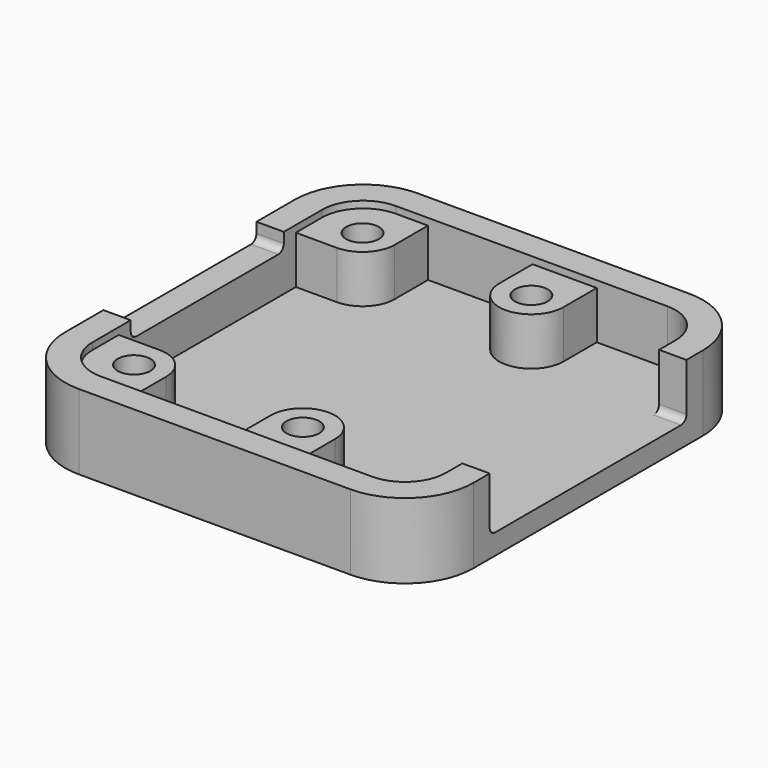
from build123d import *

# Parameters (mm, degrees)
F0_R      = 1.2
F1_DEPTH  = 1.5
F2_DEPTH  = 5
F3_DEPTH  = 5.5
F5_DEPTH  = 2
F7_DEPTH  = 2
F8_W      = 10
F8_H      = 5
F9_DEPTH  = 1
F10_R     = 1
F11_DEPTH = 5


# Not quite as in the source:
# - a feature names something its author has since deleted; it is built from what else it names


with BuildPart() as f1:
    # F0 (on Top) → F1 (new body)
    with BuildSketch(Plane.XY):
        with BuildLine():
            Line((14.9310000289, -10.5), (14.9310000289, 10.5))
            ThreePointArc((14.9310000289, 10.5), (13.4665339264, 14.0355339264), (9.931, 15.5000000289))
            Line((9.931, 15.5000000289), (-9.931, 15.5000000289))
            ThreePointArc((-9.931, 15.5000000289), (-13.4665339264, 14.0355339264), (-14.9310000289, 10.5))
            Line((-14.9310000289, 10.5), (-14.9310000289, -10.5))
            ThreePointArc((-14.9310000289, -10.5), (-13.4665339264, -14.0355339264), (-9.931, -15.5000000289))
            Line((-9.931, -15.5000000289), (9.931, -15.5000000289))
            ThreePointArc((9.931, -15.5000000289), (13.4665339264, -14.0355339264), (14.9310000289, -10.5))
        make_face()
        with BuildLine():
            Line((-9.931, 13.5000000289), (-7.581, 13.5000000289))
            Line((-7.581, 13.5000000289), (0.069, 13.5000000289))
            Line((0.069, 13.5000000289), (4.769, 13.5000000289))
            Line((4.769, 13.5000000289), (9.931, 13.5000000289))
            ThreePointArc((9.931, 13.5000000289), (12.052320364, 12.621320364), (12.9310000289, 10.5))
            Line((12.9310000289, 10.5), (12.9310000289, -10.5))
            ThreePointArc((12.9310000289, -10.5), (12.052320364, -12.621320364), (9.931, -13.5000000289))
            Line((9.931, -13.5000000289), (4.769, -13.5000000289))
            Line((4.769, -13.5000000289), (0.069, -13.5000000289))
            Line((0.069, -13.5000000289), (-7.581, -13.5000000289))
            Line((-7.581, -13.5000000289), (-9.931, -13.5000000289))
            ThreePointArc((-9.931, -13.5000000289), (-12.052320364, -12.621320364), (-12.9310000289, -10.5))
            Line((-12.9310000289, -10.5), (-12.9310000289, -8.1))
            Line((-12.9310000289, -8.1), (-12.9310000289, 8.1))
            Line((-12.9310000289, 8.1), (-12.9310000289, 10.5))
            ThreePointArc((-12.9310000289, 10.5), (-12.052320364, 12.621320364), (-9.931, 13.5000000289))
        make_face(mode=Mode.SUBTRACT)
        with BuildLine():
            ThreePointArc((4.769, -10.45), (2.419, -8.1), (0.069, -10.45))
            ThreePointArc((0.069, -10.45), (2.419, -12.8), (4.769, -10.45))
        make_face()
        with Locations((2.419, -10.45)):
            Circle(F0_R, mode=Mode.SUBTRACT)
        with BuildLine():
            ThreePointArc((4.769, 10.45), (2.419, 12.8), (0.069, 10.45))
            ThreePointArc((0.069, 10.45), (2.419, 8.1), (4.769, 10.45))
        make_face()
        with Locations((2.419, 10.45)):
            Circle(F0_R, mode=Mode.SUBTRACT)
        with BuildLine():
            ThreePointArc((-9.931, 8.1), (-11.5927009358, 12.1117009358), (-7.581, 10.45))
            Line((-7.581, 10.45), (-7.581, 13.5000000289))
            Line((-7.581, 13.5000000289), (-9.931, 13.5000000289))
            ThreePointArc((-9.931, 13.5000000289), (-12.052320364, 12.621320364), (-12.9310000289, 10.5))
            Line((-12.9310000289, 10.5), (-12.9310000289, 8.1))
            Line((-12.9310000289, 8.1), (-9.931, 8.1))
        make_face()
        with BuildLine():
            Line((-9.931, -8.1), (-12.9310000289, -8.1))
            Line((-12.9310000289, -8.1), (-12.9310000289, -10.5))
            ThreePointArc((-12.9310000289, -10.5), (-12.052320364, -12.621320364), (-9.931, -13.5000000289))
            Line((-9.931, -13.5000000289), (-7.581, -13.5000000289))
            Line((-7.581, -13.5000000289), (-7.581, -10.45))
            ThreePointArc((-7.581, -10.45), (-11.5927009358, -12.1117009358), (-9.931, -8.1))
        make_face()
        with BuildLine():
            ThreePointArc((-7.581, -10.45), (-8.2692990642, -8.7882990642), (-9.931, -8.1))
            ThreePointArc((-9.931, -8.1), (-11.5927009358, -12.1117009358), (-7.581, -10.45))
        make_face()
        with Locations((-9.931, -10.45)):
            Circle(F0_R, mode=Mode.SUBTRACT)
        with BuildLine():
            Line((0.069, -10.45), (0.069, -13.5000000289))
            Line((0.069, -13.5000000289), (4.769, -13.5000000289))
            Line((4.769, -13.5000000289), (4.769, -10.45))
            ThreePointArc((4.769, -10.45), (2.419, -12.8), (0.069, -10.45))
        make_face()
        with BuildLine():
            ThreePointArc((-9.931, 8.1), (-8.2692990642, 8.7882990642), (-7.581, 10.45))
            ThreePointArc((-7.581, 10.45), (-11.5927009358, 12.1117009358), (-9.931, 8.1))
        make_face()
        with Locations((-9.931, 10.45)):
            Circle(F0_R, mode=Mode.SUBTRACT)
        with BuildLine():
            Line((4.769, 13.5000000289), (0.069, 13.5000000289))
            Line((0.069, 13.5000000289), (0.069, 10.45))
            ThreePointArc((0.069, 10.45), (2.419, 12.8), (4.769, 10.45))
            Line((4.769, 10.45), (4.769, 13.5000000289))
        make_face()
        with BuildLine():
            Line((-7.581, 13.5000000289), (-7.581, 10.45))
            ThreePointArc((-7.581, 10.45), (-8.2692990642, 8.7882990642), (-9.931, 8.1))
            Line((-9.931, 8.1), (-12.9310000289, 8.1))
            Line((-12.9310000289, 8.1), (-12.9310000289, -8.1))
            Line((-12.9310000289, -8.1), (-9.931, -8.1))
            ThreePointArc((-9.931, -8.1), (-8.2692990642, -8.7882990642), (-7.581, -10.45))
            Line((-7.581, -10.45), (-7.581, -13.5000000289))
            Line((-7.581, -13.5000000289), (0.069, -13.5000000289))
            Line((0.069, -13.5000000289), (0.069, -10.45))
            ThreePointArc((0.069, -10.45), (2.419, -8.1), (4.769, -10.45))
            Line((4.769, -10.45), (4.769, -13.5000000289))
            Line((4.769, -13.5000000289), (9.931, -13.5000000289))
            ThreePointArc((9.931, -13.5000000289), (12.052320364, -12.621320364), (12.9310000289, -10.5))
            Line((12.9310000289, -10.5), (12.9310000289, 10.5))
            ThreePointArc((12.9310000289, 10.5), (12.052320364, 12.621320364), (9.931, 13.5000000289))
            Line((9.931, 13.5000000289), (4.769, 13.5000000289))
            Line((4.769, 13.5000000289), (4.769, 10.45))
            ThreePointArc((4.769, 10.45), (2.419, 8.1), (0.069, 10.45))
            Line((0.069, 10.45), (0.069, 13.5000000289))
            Line((0.069, 13.5000000289), (-7.581, 13.5000000289))
        make_face()
    extrude(amount=F1_DEPTH)

    # F0 (on Top) → F2 (join)
    with BuildSketch(Plane.XY):
        with BuildLine():
            ThreePointArc((-9.931, 8.1), (-11.5927009358, 12.1117009358), (-7.581, 10.45))
            Line((-7.581, 10.45), (-7.581, 13.5000000289))
            Line((-7.581, 13.5000000289), (-9.931, 13.5000000289))
            ThreePointArc((-9.931, 13.5000000289), (-12.052320364, 12.621320364), (-12.9310000289, 10.5))
            Line((-12.9310000289, 10.5), (-12.9310000289, 8.1))
            Line((-12.9310000289, 8.1), (-9.931, 8.1))
        make_face()
        with BuildLine():
            ThreePointArc((-9.931, 8.1), (-8.2692990642, 8.7882990642), (-7.581, 10.45))
            ThreePointArc((-7.581, 10.45), (-11.5927009358, 12.1117009358), (-9.931, 8.1))
        make_face()
        with Locations((-9.931, 10.45)):
            Circle(F0_R, mode=Mode.SUBTRACT)
        with BuildLine():
            ThreePointArc((4.769, 10.45), (2.419, 12.8), (0.069, 10.45))
            ThreePointArc((0.069, 10.45), (2.419, 8.1), (4.769, 10.45))
        make_face()
        with Locations((2.419, 10.45)):
            Circle(F0_R, mode=Mode.SUBTRACT)
        with BuildLine():
            Line((4.769, 13.5000000289), (0.069, 13.5000000289))
            Line((0.069, 13.5000000289), (0.069, 10.45))
            ThreePointArc((0.069, 10.45), (2.419, 12.8), (4.769, 10.45))
            Line((4.769, 10.45), (4.769, 13.5000000289))
        make_face()
        with BuildLine():
            ThreePointArc((4.769, -10.45), (2.419, -8.1), (0.069, -10.45))
            ThreePointArc((0.069, -10.45), (2.419, -12.8), (4.769, -10.45))
        make_face()
        with Locations((2.419, -10.45)):
            Circle(F0_R, mode=Mode.SUBTRACT)
        with BuildLine():
            Line((0.069, -10.45), (0.069, -13.5000000289))
            Line((0.069, -13.5000000289), (4.769, -13.5000000289))
            Line((4.769, -13.5000000289), (4.769, -10.45))
            ThreePointArc((4.769, -10.45), (2.419, -12.8), (0.069, -10.45))
        make_face()
        with BuildLine():
            ThreePointArc((-7.581, -10.45), (-8.2692990642, -8.7882990642), (-9.931, -8.1))
            ThreePointArc((-9.931, -8.1), (-11.5927009358, -12.1117009358), (-7.581, -10.45))
        make_face()
        with Locations((-9.931, -10.45)):
            Circle(F0_R, mode=Mode.SUBTRACT)
        with BuildLine():
            Line((-9.931, -8.1), (-12.9310000289, -8.1))
            Line((-12.9310000289, -8.1), (-12.9310000289, -10.5))
            ThreePointArc((-12.9310000289, -10.5), (-12.052320364, -12.621320364), (-9.931, -13.5000000289))
            Line((-9.931, -13.5000000289), (-7.581, -13.5000000289))
            Line((-7.581, -13.5000000289), (-7.581, -10.45))
            ThreePointArc((-7.581, -10.45), (-11.5927009358, -12.1117009358), (-9.931, -8.1))
        make_face()
    extrude(amount=F2_DEPTH)

    # F0 (on Top) → F3 (join)
    with BuildSketch(Plane.XY):
        with BuildLine():
            Line((14.9310000289, -10.5), (14.9310000289, 10.5))
            ThreePointArc((14.9310000289, 10.5), (13.4665339264, 14.0355339264), (9.931, 15.5000000289))
            Line((9.931, 15.5000000289), (-9.931, 15.5000000289))
            ThreePointArc((-9.931, 15.5000000289), (-13.4665339264, 14.0355339264), (-14.9310000289, 10.5))
            Line((-14.9310000289, 10.5), (-14.9310000289, -10.5))
            ThreePointArc((-14.9310000289, -10.5), (-13.4665339264, -14.0355339264), (-9.931, -15.5000000289))
            Line((-9.931, -15.5000000289), (9.931, -15.5000000289))
            ThreePointArc((9.931, -15.5000000289), (13.4665339264, -14.0355339264), (14.9310000289, -10.5))
        make_face()
        with BuildLine():
            Line((-9.931, 13.5000000289), (-7.581, 13.5000000289))
            Line((-7.581, 13.5000000289), (0.069, 13.5000000289))
            Line((0.069, 13.5000000289), (4.769, 13.5000000289))
            Line((4.769, 13.5000000289), (9.931, 13.5000000289))
            ThreePointArc((9.931, 13.5000000289), (12.052320364, 12.621320364), (12.9310000289, 10.5))
            Line((12.9310000289, 10.5), (12.9310000289, -10.5))
            ThreePointArc((12.9310000289, -10.5), (12.052320364, -12.621320364), (9.931, -13.5000000289))
            Line((9.931, -13.5000000289), (4.769, -13.5000000289))
            Line((4.769, -13.5000000289), (0.069, -13.5000000289))
            Line((0.069, -13.5000000289), (-7.581, -13.5000000289))
            Line((-7.581, -13.5000000289), (-9.931, -13.5000000289))
            ThreePointArc((-9.931, -13.5000000289), (-12.052320364, -12.621320364), (-12.9310000289, -10.5))
            Line((-12.9310000289, -10.5), (-12.9310000289, -8.1))
            Line((-12.9310000289, -8.1), (-12.9310000289, 8.1))
            Line((-12.9310000289, 8.1), (-12.9310000289, 10.5))
            ThreePointArc((-12.9310000289, 10.5), (-12.052320364, 12.621320364), (-9.931, 13.5000000289))
        make_face(mode=Mode.SUBTRACT)
    extrude(amount=F3_DEPTH)

    # F4 (on face) → F5 (cut)
    with BuildSketch(Plane(origin=(-14.9310000289, 0, 0), x_dir=(0, -1, 0), z_dir=(-1, 0, 0))):
        with BuildLine():
            Line((7, 5.5), (-7, 5.5))
            Line((-7, 5.5), (-7, 4.75))
            ThreePointArc((-7, 4.75), (-6.8535533906, 4.3964466094), (-6.5, 4.25))
            Line((-6.5, 4.25), (6.5, 4.25))
            ThreePointArc((6.5, 4.25), (6.8535533906, 4.3964466094), (7, 4.75))
            Line((7, 4.75), (7, 5.5))
        make_face()
    extrude(amount=-F5_DEPTH, mode=Mode.SUBTRACT)

    # F6 (on face) → F7 (cut)
    with BuildSketch(Plane.YZ.offset(14.9310000289)):
        with BuildLine():
            Line((9, 2), (9, 5.5))
            Line((9, 5.5), (-9, 5.5))
            Line((-9, 5.5), (-9, 2))
            ThreePointArc((-9, 2), (-8.8535533906, 1.6464466094), (-8.5, 1.5))
            Line((-8.5, 1.5), (8.5, 1.5))
            ThreePointArc((8.5, 1.5), (8.8535533906, 1.6464466094), (9, 2))
        make_face()
    extrude(amount=-F7_DEPTH, mode=Mode.SUBTRACT)

    # F8 (on face) → F9 (join)
    with BuildSketch(Plane.XY):
        Rectangle(F8_W, F8_H)
    extrude(amount=-F9_DEPTH)

    # F10 (on face) → F11 (join)
    with BuildSketch(Plane(origin=(0, 2.5, 0), x_dir=(-1, 0, 0), z_dir=(0, 1, 0))):
        with BuildLine():
            Line((5, -1), (-5, -1))
            ThreePointArc((-5, -1), (0, -6), (5, -1))
        make_face()
        with Locations((0, -4)):
            Circle(F10_R, mode=Mode.SUBTRACT)
    extrude(amount=-F11_DEPTH)


solid = f1.part
